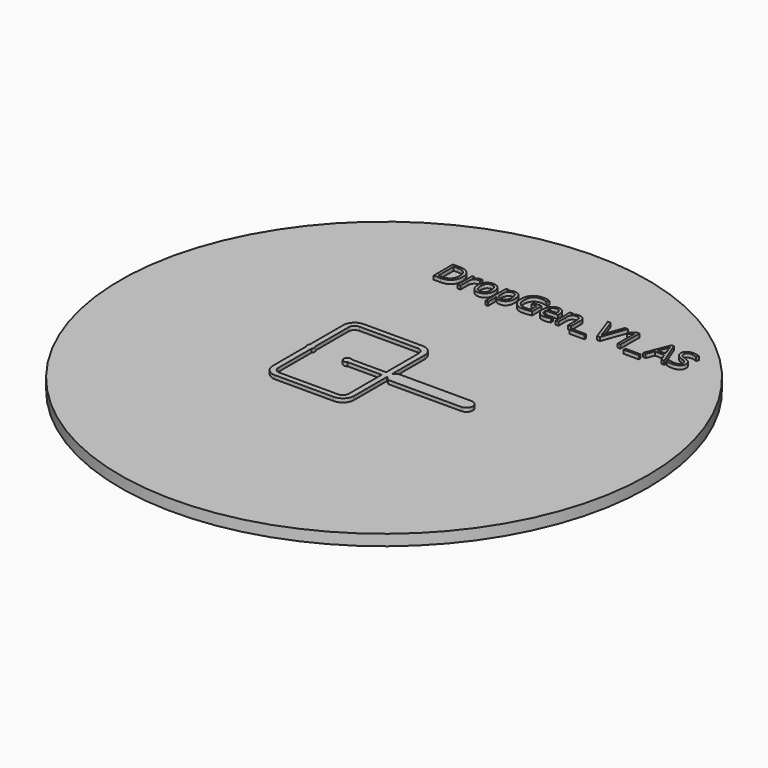
from build123d import *

# Parameters (mm, degrees)
F0_R         = 36
F0_W         = 2.0741813148
F0_H         = 0.2931375804
F0_TEXT_SIZE = 4.5869939236
F1_DEPTH     = 1.5
F2_DEPTH     = 0.5


# Not quite as in the source:
# - Text() gives the source's letters only with a copy of the font that has no kerning and outlines rounded to 1/6400 em; it was checked with that copy


with BuildPart() as f1:
    # F0 (on Top) → F1 (new body)
    with BuildSketch(Plane.XY):
        Circle(F0_R)
        with BuildLine():
            add(Edge.make_bspline(
                [(-6.0150917545, 23.3154267102), (-5.8222946662, 23.445510991), (-5.5915115344, 23.445510991)],
                knots=[0, 0, 0, 1, 1, 1], degree=2))
            add(Edge.make_bspline(
                [(-5.5915115344, 23.445510991), (-5.4280998758, 23.445510991), (-5.2983739539, 23.4182757146)],
                knots=[0, 0, 0, 1, 1, 1], degree=2))
            Line((-5.2983739539, 23.4182757146), (-5.3499776356, 23.0735344525))
            add(Edge.make_bspline(
                [(-5.3499776356, 23.0735344525), (-5.5019218093, 23.1072201892), (-5.6187468108, 23.1072201892)],
                knots=[0, 0, 0, 1, 1, 1], degree=2))
            add(Edge.make_bspline(
                [(-5.6187468108, 23.1072201892), (-5.9169014158, 23.1072201892), (-6.128333167, 22.8653279315)],
                knots=[0, 0, 0, 1, 1, 1], degree=2))
            add(Edge.make_bspline(
                [(-6.128333167, 22.8653279315), (-6.3397649182, 22.6234356738), (-6.3397649182, 22.2629266201)],
                knots=[0, 0, 0, 1, 1, 1], degree=2))
            Line((-6.3397649182, 22.2629266201), (-6.3397649182, 20.9455993026))
            Line((-6.3397649182, 20.9455993026), (-6.7117414567, 20.9455993026))
            Line((-6.7117414567, 20.9455993026), (-6.7117414567, 23.4003577696))
            Line((-6.7117414567, 23.4003577696), (-6.404986238, 23.4003577696))
            Line((-6.404986238, 23.4003577696), (-6.36198317, 22.945958684))
            Line((-6.36198317, 22.945958684), (-6.344065225, 22.945958684))
            add(Edge.make_bspline(
                [(-6.344065225, 22.945958684), (-6.2078888429, 23.1853424294), (-6.0150917545, 23.3154267102)],
                knots=[0, 0, 0, 1, 1, 1], degree=2))
        make_face(mode=Mode.SUBTRACT)
        with BuildLine():
            add(Edge.make_bspline(
                [(-3.0238700138, 23.1025615235), (-2.7203400253, 22.7596120559), (-2.7203400253, 22.1754870484)],
                knots=[0, 0, 0, 1, 1, 1], degree=2))
            add(Edge.make_bspline(
                [(-2.7203400253, 22.1754870484), (-2.7203400253, 21.5748775315), (-3.0224365782, 21.2376618064)],
                knots=[0, 0, 0, 1, 1, 1], degree=2))
            add(Edge.make_bspline(
                [(-3.0224365782, 21.2376618064), (-3.3245331312, 20.9004460812), (-3.8577711748, 20.9004460812)],
                knots=[0, 0, 0, 1, 1, 1], degree=2))
            add(Edge.make_bspline(
                [(-3.8577711748, 20.9004460812), (-4.1874613631, 20.9004460812), (-4.4426129001, 21.0552571261)],
                knots=[0, 0, 0, 1, 1, 1], degree=2))
            add(Edge.make_bspline(
                [(-4.4426129001, 21.0552571261), (-4.6977644371, 21.2100681711), (-4.8368076904, 21.4989054447)],
                knots=[0, 0, 0, 1, 1, 1], degree=2))
            add(Edge.make_bspline(
                [(-4.8368076904, 21.4989054447), (-4.9758509437, 21.7877427183), (-4.9758509437, 22.1754870484)],
                knots=[0, 0, 0, 1, 1, 1], degree=2))
            add(Edge.make_bspline(
                [(-4.9758509437, 22.1754870484), (-4.9758509437, 22.7753798475), (-4.6755461853, 23.1104454193)],
                knots=[0, 0, 0, 1, 1, 1], degree=2))
            add(Edge.make_bspline(
                [(-4.6755461853, 23.1104454193), (-4.3752414268, 23.445510991), (-3.8420033832, 23.445510991)],
                knots=[0, 0, 0, 1, 1, 1], degree=2))
            add(Edge.make_bspline(
                [(-3.8420033832, 23.445510991), (-3.3274000024, 23.445510991), (-3.0238700138, 23.1025615235)],
                knots=[0, 0, 0, 1, 1, 1], degree=2))
        make_face(mode=Mode.SUBTRACT)
        with BuildLine():
            add(Edge.make_bspline(
                [(-0.1763501922, 21.235511653), (-0.4461944441, 20.9004460812), (-0.9256786527, 20.9004460812)],
                knots=[0, 0, 0, 1, 1, 1], degree=2))
            add(Edge.make_bspline(
                [(-0.9256786527, 20.9004460812), (-1.1657791159, 20.9004460812), (-1.3639515877, 20.9889607296)],
                knots=[0, 0, 0, 1, 1, 1], degree=2))
            add(Edge.make_bspline(
                [(-1.3639515877, 20.9889607296), (-1.5621240596, 21.077475378), (-1.6961502883, 21.2616718527)],
                knots=[0, 0, 0, 1, 1, 1], degree=2))
            Line((-1.6961502883, 21.2616718527), (-1.7233855647, 21.2616718527))
            add(Edge.make_bspline(
                [(-1.7233855647, 21.2616718527), (-1.6961502883, 21.0466565125), (-1.6961502883, 20.8538594242)],
                knots=[0, 0, 0, 1, 1, 1], degree=2))
            Line((-1.6961502883, 20.8538594242), (-1.6961502883, 19.8432873254))
            Line((-1.6961502883, 19.8432873254), (-2.0681268268, 19.8432873254))
            Line((-2.0681268268, 19.8432873254), (-2.0681268268, 23.4003577696))
            Line((-2.0681268268, 23.4003577696), (-1.765671915, 23.4003577696))
            Line((-1.765671915, 23.4003577696), (-1.7140682333, 23.0642171211))
            Line((-1.7140682333, 23.0642171211), (-1.6961502883, 23.0642171211))
            add(Edge.make_bspline(
                [(-1.6961502883, 23.0642171211), (-1.5528067282, 23.2663315409), (-1.3625181521, 23.355921266)],
                knots=[0, 0, 0, 1, 1, 1], degree=2))
            add(Edge.make_bspline(
                [(-1.3625181521, 23.355921266), (-1.1722295761, 23.445510991), (-0.9256786527, 23.445510991)],
                knots=[0, 0, 0, 1, 1, 1], degree=2))
            add(Edge.make_bspline(
                [(-0.9256786527, 23.445510991), (-0.4375938305, 23.445510991), (-0.1720498854, 23.111520496)],
                knots=[0, 0, 0, 1, 1, 1], degree=2))
            add(Edge.make_bspline(
                [(-0.1720498854, 23.111520496), (0.0934940597, 22.7775300009), (0.0934940597, 22.1754870484)],
                knots=[0, 0, 0, 1, 1, 1], degree=2))
            add(Edge.make_bspline(
                [(0.0934940597, 22.1754870484), (0.0934940597, 21.5705772247), (-0.1763501922, 21.235511653)],
                knots=[0, 0, 0, 1, 1, 1], degree=2))
        make_face(mode=Mode.SUBTRACT)
        with BuildLine():
            add(Edge.make_bspline(
                [(-7.8093947682, 23.7970610722), (-7.386172907, 23.373839211), (-7.386172907, 22.6141183424)],
                knots=[0, 0, 0, 1, 1, 1], degree=2))
            add(Edge.make_bspline(
                [(-7.386172907, 22.6141183424), (-7.386172907, 21.8035105099), (-7.8262376365, 21.3745549063)],
                knots=[0, 0, 0, 1, 1, 1], degree=2))
            add(Edge.make_bspline(
                [(-7.8262376365, 21.3745549063), (-8.2663023661, 20.9455993026), (-9.0926779901, 20.9455993026)],
                knots=[0, 0, 0, 1, 1, 1], degree=2))
            Line((-9.0926779901, 20.9455993026), (-10.0000427257, 20.9455993026))
            Line((-10.0000427257, 20.9455993026), (-10.0000427257, 24.2202829334))
            Line((-10.0000427257, 24.2202829334), (-8.9966378049, 24.2202829334))
            add(Edge.make_bspline(
                [(-8.9966378049, 24.2202829334), (-8.2326166295, 24.2202829334), (-7.8093947682, 23.7970610722)],
                knots=[0, 0, 0, 1, 1, 1], degree=2))
        make_face(mode=Mode.SUBTRACT)
        with BuildLine():
            Line((-10.375, 0.3307189139), (-10.375, 6))
            ThreePointArc((-10.375, 6), (-9.9210155108, 7.0960155108), (-8.825, 7.55))
            Line((-8.825, 7.55), (-0.825, 7.55))
            ThreePointArc((-0.825, 7.55), (0.2710155108, 7.0960155108), (0.725, 6))
            Line((0.725, 6), (0.725, 0.375))
            Line((0.725, 0.375), (1.225, 0.875))
            Line((1.225, 0.875), (11.225, 0.875))
            ThreePointArc((11.225, 0.875), (11.8437184335, 0.6187184335), (12.1, 0))
            ThreePointArc((12.1, 0), (11.8437184335, -0.6187184335), (11.225, -0.875))
            Line((11.225, -0.875), (1.225, -0.875))
            Line((1.225, -0.875), (0.725, -0.375))
            Line((0.725, -0.375), (0.725, -6))
            ThreePointArc((0.725, -6), (0.2710155108, -7.0960155108), (-0.825, -7.55))
            Line((-0.825, -7.55), (-8.825, -7.55))
            ThreePointArc((-8.825, -7.55), (-9.9210155108, -7.0960155108), (-10.375, -6))
            Line((-10.375, -6), (-10.375, -0.3307189139))
            ThreePointArc((-10.375, -0.3307189139), (-10.5, 0), (-10.375, 0.3307189139))
        make_face(mode=Mode.SUBTRACT)
        with BuildLine():
            add(Edge.make_bspline(
                [(5.5434162152, 20.9377154068), (5.3678203541, 20.9004460812), (5.1191192773, 20.9004460812)],
                knots=[0, 0, 0, 1, 1, 1], degree=2))
            add(Edge.make_bspline(
                [(5.1191192773, 20.9004460812), (4.5751304666, 20.9004460812), (4.2601329933, 21.2322864229)],
                knots=[0, 0, 0, 1, 1, 1], degree=2))
            add(Edge.make_bspline(
                [(4.2601329933, 21.2322864229), (3.9451355199, 21.5641267645), (3.9451355199, 22.1525520788)],
                knots=[0, 0, 0, 1, 1, 1], degree=2))
            add(Edge.make_bspline(
                [(3.9451355199, 22.1525520788), (3.9451355199, 22.7467111355), (4.2375563826, 23.0961110632)],
                knots=[0, 0, 0, 1, 1, 1], degree=2))
            add(Edge.make_bspline(
                [(4.2375563826, 23.0961110632), (4.5299772452, 23.445510991), (5.023079092, 23.445510991)],
                knots=[0, 0, 0, 1, 1, 1], degree=2))
            add(Edge.make_bspline(
                [(5.023079092, 23.445510991), (5.4839286378, 23.445510991), (5.752697813, 23.1419810025)],
                knots=[0, 0, 0, 1, 1, 1], degree=2))
            add(Edge.make_bspline(
                [(5.752697813, 23.1419810025), (6.0214669882, 22.8384510139), (6.0214669882, 22.3410488604)],
                knots=[0, 0, 0, 1, 1, 1], degree=2))
            Line((6.0214669882, 22.3410488604), (6.0214669882, 22.1059654218))
            Line((6.0214669882, 22.1059654218), (4.3307296967, 22.1059654218))
            add(Edge.make_bspline(
                [(4.3307296967, 22.1059654218), (4.3421971815, 21.673784588), (4.5493286258, 21.4498102753)],
                knots=[0, 0, 0, 1, 1, 1], degree=2))
            add(Edge.make_bspline(
                [(4.5493286258, 21.4498102753), (4.7564600702, 21.2258359627), (5.1327369155, 21.2258359627)],
                knots=[0, 0, 0, 1, 1, 1], degree=2))
            add(Edge.make_bspline(
                [(5.1327369155, 21.2258359627), (5.5290818592, 21.2258359627), (5.9161094715, 21.3913977746)],
                knots=[0, 0, 0, 1, 1, 1], degree=2))
            Line((5.9161094715, 21.3913977746), (5.9161094715, 21.0595574329))
            add(Edge.make_bspline(
                [(5.9161094715, 21.0595574329), (5.7190120763, 20.9749847325), (5.5434162152, 20.9377154068)],
                knots=[0, 0, 0, 1, 1, 1], degree=2))
        make_face(mode=Mode.SUBTRACT)
        with BuildLine():
            Line((8.7077253047, 20.9455993026), (8.3357487662, 20.9455993026))
            Line((8.3357487662, 20.9455993026), (8.3357487662, 22.5338459487))
            add(Edge.make_bspline(
                [(8.3357487662, 22.5338459487), (8.3357487662, 22.8334339893), (8.1992140252, 22.9814362152)],
                knots=[0, 0, 0, 1, 1, 1], degree=2))
            add(Edge.make_bspline(
                [(8.1992140252, 22.9814362152), (8.0626792842, 23.129438441), (7.7709751394, 23.129438441)],
                knots=[0, 0, 0, 1, 1, 1], degree=2))
            add(Edge.make_bspline(
                [(7.7709751394, 23.129438441), (7.3860976805, 23.129438441), (7.2069182303, 22.9212319199)],
                knots=[0, 0, 0, 1, 1, 1], degree=2))
            add(Edge.make_bspline(
                [(7.2069182303, 22.9212319199), (7.0277387802, 22.7130253988), (7.0277387802, 22.2335411903)],
                knots=[0, 0, 0, 1, 1, 1], degree=2))
            Line((7.0277387802, 22.2335411903), (7.0277387802, 20.9455993026))
            Line((7.0277387802, 20.9455993026), (6.6557622417, 20.9455993026))
            Line((6.6557622417, 20.9455993026), (6.6557622417, 23.4003577696))
            Line((6.6557622417, 23.4003577696), (6.9582171535, 23.4003577696))
            Line((6.9582171535, 23.4003577696), (7.0184214488, 23.0642171211))
            Line((7.0184214488, 23.0642171211), (7.0363393938, 23.0642171211))
            add(Edge.make_bspline(
                [(7.0363393938, 23.0642171211), (7.1510142419, 23.2455467247), (7.3570706095, 23.3455288578)],
                knots=[0, 0, 0, 1, 1, 1], degree=2))
            add(Edge.make_bspline(
                [(7.3570706095, 23.3455288578), (7.5631269772, 23.445510991), (7.8161283608, 23.445510991)],
                knots=[0, 0, 0, 1, 1, 1], degree=2))
            add(Edge.make_bspline(
                [(7.8161283608, 23.445510991), (8.2597766793, 23.445510991), (8.483750992, 23.2315707276)],
                knots=[0, 0, 0, 1, 1, 1], degree=2))
            add(Edge.make_bspline(
                [(8.483750992, 23.2315707276), (8.7077253047, 23.0176304641), (8.7077253047, 22.5467468691)],
                knots=[0, 0, 0, 1, 1, 1], degree=2))
            Line((8.7077253047, 22.5467468691), (8.7077253047, 20.9455993026))
        make_face(mode=Mode.SUBTRACT)
        with BuildLine():
            Line((2.2393471546, 22.3209807619), (2.2393471546, 22.6614217172))
            Line((2.2393471546, 22.6614217172), (3.3524098989, 22.6614217172))
            Line((3.3524098989, 22.6614217172), (3.3524098989, 21.0688747643))
            add(Edge.make_bspline(
                [(3.3524098989, 21.0688747643), (3.0922413373, 20.9857354995), (2.8234721621, 20.9430907903)],
                knots=[0, 0, 0, 1, 1, 1], degree=2))
            add(Edge.make_bspline(
                [(2.8234721621, 20.9430907903), (2.5547029869, 20.9004460812), (2.2006443934, 20.9004460812)],
                knots=[0, 0, 0, 1, 1, 1], degree=2))
            add(Edge.make_bspline(
                [(2.2006443934, 20.9004460812), (1.4574080342, 20.9004460812), (1.0431451455, 21.3430193231)],
                knots=[0, 0, 0, 1, 1, 1], degree=2))
            add(Edge.make_bspline(
                [(1.0431451455, 21.3430193231), (0.6288822567, 21.7855925649), (0.6288822567, 22.5825827591)],
                knots=[0, 0, 0, 1, 1, 1], degree=2))
            add(Edge.make_bspline(
                [(0.6288822567, 22.5825827591), (0.6288822567, 23.0936025509), (0.8338635477, 23.477763292)],
                knots=[0, 0, 0, 1, 1, 1], degree=2))
            add(Edge.make_bspline(
                [(0.8338635477, 23.477763292), (1.0388448387, 23.8619240331), (1.4240806565, 24.0643968118)],
                knots=[0, 0, 0, 1, 1, 1], degree=2))
            add(Edge.make_bspline(
                [(1.4240806565, 24.0643968118), (1.8093164743, 24.2668695905), (2.3260700085, 24.2668695905)],
                knots=[0, 0, 0, 1, 1, 1], degree=2))
            add(Edge.make_bspline(
                [(2.3260700085, 24.2668695905), (2.8507074385, 24.2668695905), (3.3029563706, 24.0747892199)],
                knots=[0, 0, 0, 1, 1, 1], degree=2))
            Line((3.3029563706, 24.0747892199), (3.1553125037, 23.7386485715))
            add(Edge.make_bspline(
                [(3.1553125037, 23.7386485715), (2.7116641852, 23.9264286352), (2.3017016033, 23.9264286352)],
                knots=[0, 0, 0, 1, 1, 1], degree=2))
            add(Edge.make_bspline(
                [(2.3017016033, 23.9264286352), (1.7039589576, 23.9264286352), (1.3678183091, 23.5705782472)],
                knots=[0, 0, 0, 1, 1, 1], degree=2))
            add(Edge.make_bspline(
                [(1.3678183091, 23.5705782472), (1.0316776606, 23.2147278592), (1.0316776606, 22.5825827591)],
                knots=[0, 0, 0, 1, 1, 1], degree=2))
            add(Edge.make_bspline(
                [(1.0316776606, 22.5825827591), (1.0316776606, 21.9196187936), (1.3552757476, 21.5770276849)],
                knots=[0, 0, 0, 1, 1, 1], degree=2))
            add(Edge.make_bspline(
                [(1.3552757476, 21.5770276849), (1.6788738346, 21.2344365763), (2.3060019101, 21.2344365763)],
                knots=[0, 0, 0, 1, 1, 1], degree=2))
            add(Edge.make_bspline(
                [(2.3060019101, 21.2344365763), (2.6464428653, 21.2344365763), (2.971116029, 21.3132755343)],
                knots=[0, 0, 0, 1, 1, 1], degree=2))
            Line((2.971116029, 21.3132755343), (2.971116029, 22.3209807619))
            Line((2.971116029, 22.3209807619), (2.2393471546, 22.3209807619))
        make_face(mode=Mode.SUBTRACT)
        with Locations((10.104608298, 20.3869177771)):
            Rectangle(F0_W, F0_H, mode=Mode.SUBTRACT)
        with Locations((17.5133202024, 20.3869177771)):
            Rectangle(F0_W, F0_H, mode=Mode.SUBTRACT)
        with BuildLine():
            Line((12.7055771963, 22.1145660354), (13.45383058, 24.2202829334))
            Line((13.45383058, 24.2202829334), (13.8630764442, 24.2202829334))
            Line((13.8630764442, 24.2202829334), (12.6833589444, 20.9455993026))
            Line((12.6833589444, 20.9455993026), (12.3070820991, 20.9455993026))
            Line((12.3070820991, 20.9455993026), (11.1330983418, 24.2202829334))
            Line((11.1330983418, 24.2202829334), (11.5366104635, 24.2202829334))
            Line((11.5366104635, 24.2202829334), (12.2891641541, 22.101665115))
            add(Edge.make_bspline(
                [(12.2891641541, 22.101665115), (12.418890076, 21.7361390367), (12.4948621629, 21.3913977746)],
                knots=[0, 0, 0, 1, 1, 1], degree=2))
            add(Edge.make_bspline(
                [(12.4948621629, 21.3913977746), (12.5758512744, 21.7540569817), (12.7055771963, 22.1145660354)],
                knots=[0, 0, 0, 1, 1, 1], degree=2))
        make_face(mode=Mode.SUBTRACT)
        with BuildLine():
            Line((15.4642240106, 24.2202829334), (15.4642240106, 20.9455993026))
            Line((15.4642240106, 20.9455993026), (15.1015648035, 20.9455993026))
            Line((15.1015648035, 20.9455993026), (15.1015648035, 23.2792324613))
            add(Edge.make_bspline(
                [(15.1015648035, 23.2792324613), (15.1015648035, 23.5709366061), (15.1194827486, 23.8303884499)],
                knots=[0, 0, 0, 1, 1, 1], degree=2))
            add(Edge.make_bspline(
                [(15.1194827486, 23.8303884499), (15.0728960915, 23.7830850751), (15.0144835908, 23.7318397523)],
                knots=[0, 0, 0, 1, 1, 1], degree=2))
            add(Edge.make_bspline(
                [(15.0144835908, 23.7318397523), (14.95607109, 23.6805944296), (14.4816039061, 23.2950002529)],
                knots=[0, 0, 0, 1, 1, 1], degree=2))
            Line((14.4816039061, 23.2950002529), (14.2845065109, 23.5501517899))
            Line((14.2845065109, 23.5501517899), (15.1510183318, 24.2202829334))
            Line((15.1510183318, 24.2202829334), (15.4642240106, 24.2202829334))
        make_face(mode=Mode.SUBTRACT)
        Polygon((21.4445173385, 20.9455993026), (21.0503225482, 20.9455993026), (20.6425101197, 21.9869902669), (19.3301998269, 21.9869902669), (18.927404423, 20.9455993026), (18.5418102463, 20.9455993026), (19.8362025941, 24.2339005716), (20.1565754509, 24.2339005716), align=None, mode=Mode.SUBTRACT)
        with BuildLine():
            add(Edge.make_bspline(
                [(23.548800801, 22.3632671122), (23.7423146072, 22.1525520788), (23.7423146072, 21.8171281481)],
                knots=[0, 0, 0, 1, 1, 1], degree=2))
            add(Edge.make_bspline(
                [(23.7423146072, 21.8171281481), (23.7423146072, 21.3849473144), (23.4287505694, 21.1426966978)],
                knots=[0, 0, 0, 1, 1, 1], degree=2))
            add(Edge.make_bspline(
                [(23.4287505694, 21.1426966978), (23.1151865317, 20.9004460812), (22.5776481812, 20.9004460812)],
                knots=[0, 0, 0, 1, 1, 1], degree=2))
            add(Edge.make_bspline(
                [(22.5776481812, 20.9004460812), (21.9956733272, 20.9004460812), (21.6817509305, 21.0509568193)],
                knots=[0, 0, 0, 1, 1, 1], degree=2))
            Line((21.6817509305, 21.0509568193), (21.6817509305, 21.4179163332))
            add(Edge.make_bspline(
                [(21.6817509305, 21.4179163332), (21.8838653503, 21.3333436328), (22.1210989423, 21.2838901045)],
                knots=[0, 0, 0, 1, 1, 1], degree=2))
            add(Edge.make_bspline(
                [(22.1210989423, 21.2838901045), (22.3583325343, 21.2344365763), (22.5912658195, 21.2344365763)],
                knots=[0, 0, 0, 1, 1, 1], degree=2))
            add(Edge.make_bspline(
                [(22.5912658195, 21.2344365763), (22.9718429716, 21.2344365763), (23.1646400599, 21.3788552131)],
                knots=[0, 0, 0, 1, 1, 1], degree=2))
            add(Edge.make_bspline(
                [(23.1646400599, 21.3788552131), (23.3574371483, 21.5232738499), (23.3574371483, 21.7812922581)],
                knots=[0, 0, 0, 1, 1, 1], degree=2))
            add(Edge.make_bspline(
                [(23.3574371483, 21.7812922581), (23.3574371483, 21.9511543768), (23.2889905983, 22.0597371236)],
                knots=[0, 0, 0, 1, 1, 1], degree=2))
            add(Edge.make_bspline(
                [(23.2889905983, 22.0597371236), (23.2205440483, 22.1683198704), (23.0603576199, 22.2604181078)],
                knots=[0, 0, 0, 1, 1, 1], degree=2))
            add(Edge.make_bspline(
                [(23.0603576199, 22.2604181078), (22.9001711915, 22.3525163452), (22.5733478744, 22.4686246289)],
                knots=[0, 0, 0, 1, 1, 1], degree=2))
            add(Edge.make_bspline(
                [(22.5733478744, 22.4686246289), (22.1167986355, 22.6320362874), (21.920776317, 22.8560106001)],
                knots=[0, 0, 0, 1, 1, 1], degree=2))
            add(Edge.make_bspline(
                [(21.920776317, 22.8560106001), (21.7247539986, 23.0799849127), (21.7247539986, 23.4404939664)],
                knots=[0, 0, 0, 1, 1, 1], degree=2))
            add(Edge.make_bspline(
                [(21.7247539986, 23.4404939664), (21.7247539986, 23.8189209651), (22.0089326065, 24.0428952778)],
                knots=[0, 0, 0, 1, 1, 1], degree=2))
            add(Edge.make_bspline(
                [(22.0089326065, 24.0428952778), (22.2931112144, 24.2668695905), (22.761844656, 24.2668695905)],
                knots=[0, 0, 0, 1, 1, 1], degree=2))
            add(Edge.make_bspline(
                [(22.761844656, 24.2668695905), (23.2499294782, 24.2668695905), (23.6598920601, 24.0876901403)],
                knots=[0, 0, 0, 1, 1, 1], degree=2))
            Line((23.6598920601, 24.0876901403), (23.5409169052, 23.7565665165))
            add(Edge.make_bspline(
                [(23.5409169052, 23.7565665165), (23.1352546301, 23.9264286352), (22.7525273246, 23.9264286352)],
                knots=[0, 0, 0, 1, 1, 1], degree=2))
            add(Edge.make_bspline(
                [(22.7525273246, 23.9264286352), (22.4500724127, 23.9264286352), (22.2798519351, 23.7967027133)],
                knots=[0, 0, 0, 1, 1, 1], degree=2))
            add(Edge.make_bspline(
                [(22.2798519351, 23.7967027133), (22.1096314575, 23.6669767914), (22.1096314575, 23.4361936596)],
                knots=[0, 0, 0, 1, 1, 1], degree=2))
            add(Edge.make_bspline(
                [(22.1096314575, 23.4361936596), (22.1096314575, 23.2663315409), (22.172344265, 23.1573904352)],
                knots=[0, 0, 0, 1, 1, 1], degree=2))
            add(Edge.make_bspline(
                [(22.172344265, 23.1573904352), (22.2350570726, 23.0484493295), (22.3841343751, 22.9577845277)],
                knots=[0, 0, 0, 1, 1, 1], degree=2))
            add(Edge.make_bspline(
                [(22.3841343751, 22.9577845277), (22.5332116776, 22.867119726), (22.8399668962, 22.7574619025)],
                knots=[0, 0, 0, 1, 1, 1], degree=2))
            add(Edge.make_bspline(
                [(22.8399668962, 22.7574619025), (23.3552869949, 22.5739821455), (23.548800801, 22.3632671122)],
                knots=[0, 0, 0, 1, 1, 1], degree=2))
        make_face(mode=Mode.SUBTRACT)
        with BuildLine():
            ThreePointArc((-8.825, 7.55), (-9.9210155108, 7.0960155108), (-10.375, 6))
            Line((-10.375, 6), (-10.375, 0.3307189139))
            ThreePointArc((-10.375, 0.3307189139), (-10.5, 0), (-10.375, -0.3307189139))
            Line((-10.375, -0.3307189139), (-10.375, -6))
            ThreePointArc((-10.375, -6), (-9.9210155108, -7.0960155108), (-8.825, -7.55))
            Line((-8.825, -7.55), (-0.825, -7.55))
            ThreePointArc((-0.825, -7.55), (0.2710155108, -7.0960155108), (0.725, -6))
            Line((0.725, -6), (0.725, -0.375))
            Line((0.725, -0.375), (1.225, -0.875))
            Line((1.225, -0.875), (11.225, -0.875))
            ThreePointArc((11.225, -0.875), (10.35, 0), (11.225, 0.875))
            Line((11.225, 0.875), (1.225, 0.875))
            Line((1.225, 0.875), (0.725, 0.375))
            Line((0.725, 0.375), (0.725, 6))
            ThreePointArc((0.725, 6), (0.2710155108, 7.0960155108), (-0.825, 7.55))
            Line((-0.825, 7.55), (-8.825, 7.55))
        make_face()
        with BuildLine():
            Line((-9.625, 0.3307189139), (-9.625, 6))
            ThreePointArc((-9.625, 6), (-9.3906854249, 6.5656854249), (-8.825, 6.8))
            Line((-8.825, 6.8), (-0.825, 6.8))
            ThreePointArc((-0.825, 6.8), (-0.2593145751, 6.5656854249), (-0.025, 6))
            Line((-0.025, 6), (-0.025, 0.375))
            Line((-0.025, 0.375), (-4.6692810861, 0.375))
            ThreePointArc((-4.6692810861, 0.375), (-5.5, 0), (-4.6692810861, -0.375))
            Line((-4.6692810861, -0.375), (-0.025, -0.375))
            Line((-0.025, -0.375), (-0.025, -6))
            ThreePointArc((-0.025, -6), (-0.2593145751, -6.5656854249), (-0.825, -6.8))
            Line((-0.825, -6.8), (-8.825, -6.8))
            ThreePointArc((-8.825, -6.8), (-9.3906854249, -6.5656854249), (-9.625, -6))
            Line((-9.625, -6), (-9.625, -0.3307189139))
            ThreePointArc((-9.625, -0.3307189139), (-9.5, 0), (-9.625, 0.3307189139))
        make_face(mode=Mode.SUBTRACT)
        with BuildLine():
            ThreePointArc((-8.825, 6.8), (-9.3906854249, 6.5656854249), (-9.625, 6))
            Line((-9.625, 6), (-9.625, 0.3307189139))
            ThreePointArc((-9.625, 0.3307189139), (-9.5, 0), (-9.625, -0.3307189139))
            Line((-9.625, -0.3307189139), (-9.625, -6))
            ThreePointArc((-9.625, -6), (-9.3906854249, -6.5656854249), (-8.825, -6.8))
            Line((-8.825, -6.8), (-0.825, -6.8))
            ThreePointArc((-0.825, -6.8), (-0.2593145751, -6.5656854249), (-0.025, -6))
            Line((-0.025, -6), (-0.025, -0.375))
            Line((-0.025, -0.375), (-4.6692810861, -0.375))
            ThreePointArc((-4.6692810861, -0.375), (-5.5, 0), (-4.6692810861, 0.375))
            Line((-4.6692810861, 0.375), (-0.025, 0.375))
            Line((-0.025, 0.375), (-0.025, 6))
            ThreePointArc((-0.025, 6), (-0.2593145751, 6.5656854249), (-0.825, 6.8))
            Line((-0.825, 6.8), (-8.825, 6.8))
        make_face()
        with BuildLine():
            add(Edge.make_bspline(
                [(-8.1319177785, 21.6096383449), (-7.7889683109, 21.9447039166), (-7.7889683109, 22.6005007042)],
                knots=[0, 0, 0, 1, 1, 1], degree=2))
            add(Edge.make_bspline(
                [(-7.7889683109, 22.6005007042), (-7.7889683109, 23.2412464179), (-8.1104162445, 23.5659195815)],
                knots=[0, 0, 0, 1, 1, 1], degree=2))
            add(Edge.make_bspline(
                [(-8.1104162445, 23.5659195815), (-8.431864178, 23.8905927452), (-9.0661594315, 23.8905927452)],
                knots=[0, 0, 0, 1, 1, 1], degree=2))
            Line((-9.0661594315, 23.8905927452), (-9.6194655736, 23.8905927452))
            Line((-9.6194655736, 23.8905927452), (-9.6194655736, 21.2745727731))
            Line((-9.6194655736, 21.2745727731), (-9.1557491566, 21.2745727731))
            add(Edge.make_bspline(
                [(-9.1557491566, 21.2745727731), (-8.474867246, 21.2745727731), (-8.1319177785, 21.6096383449)],
                knots=[0, 0, 0, 1, 1, 1], degree=2))
        make_face()
        with BuildLine():
            ThreePointArc((12.1, 0), (11.8437184335, 0.6187184335), (11.225, 0.875))
            ThreePointArc((11.225, 0.875), (10.35, 0), (11.225, -0.875))
            ThreePointArc((11.225, -0.875), (11.8437184335, -0.6187184335), (12.1, 0))
        make_face()
        with BuildLine():
            add(Edge.make_bspline(
                [(-4.4042684977, 22.8896963367), (-4.590256767, 22.6499542324), (-4.590256767, 22.1754870484)],
                knots=[0, 0, 0, 1, 1, 1], degree=2))
            add(Edge.make_bspline(
                [(-4.590256767, 22.1754870484), (-4.590256767, 21.7046034534), (-4.4021183443, 21.458410889)],
                knots=[0, 0, 0, 1, 1, 1], degree=2))
            add(Edge.make_bspline(
                [(-4.4021183443, 21.458410889), (-4.2139799217, 21.2122183245), (-3.8491705612, 21.2122183245)],
                knots=[0, 0, 0, 1, 1, 1], degree=2))
            add(Edge.make_bspline(
                [(-3.8491705612, 21.2122183245), (-3.4836444829, 21.2122183245), (-3.2944309836, 21.4573358123)],
                knots=[0, 0, 0, 1, 1, 1], degree=2))
            add(Edge.make_bspline(
                [(-3.2944309836, 21.4573358123), (-3.1052174842, 21.7024533), (-3.1052174842, 22.1754870484)],
                knots=[0, 0, 0, 1, 1, 1], degree=2))
            add(Edge.make_bspline(
                [(-3.1052174842, 22.1754870484), (-3.1052174842, 22.6435037722), (-3.2944309836, 22.8864711066)],
                knots=[0, 0, 0, 1, 1, 1], degree=2))
            add(Edge.make_bspline(
                [(-3.2944309836, 22.8864711066), (-3.4836444829, 23.129438441), (-3.853470868, 23.129438441)],
                knots=[0, 0, 0, 1, 1, 1], degree=2))
            add(Edge.make_bspline(
                [(-3.853470868, 23.129438441), (-4.2182802285, 23.129438441), (-4.4042684977, 22.8896963367)],
                knots=[0, 0, 0, 1, 1, 1], degree=2))
        make_face()
        with BuildLine():
            add(Edge.make_bspline(
                [(-0.4723546438, 22.8843209532), (-0.6526091707, 23.129438441), (-0.9794324877, 23.129438441)],
                knots=[0, 0, 0, 1, 1, 1], degree=2))
            add(Edge.make_bspline(
                [(-0.9794324877, 23.129438441), (-1.355709333, 23.129438441), (-1.5237796573, 22.9212319199)],
                knots=[0, 0, 0, 1, 1, 1], degree=2))
            add(Edge.make_bspline(
                [(-1.5237796573, 22.9212319199), (-1.6918499815, 22.7130253988), (-1.6961502883, 22.2579095955)],
                knots=[0, 0, 0, 1, 1, 1], degree=2))
            Line((-1.6961502883, 22.2579095955), (-1.6961502883, 22.1754870484))
            add(Edge.make_bspline(
                [(-1.6961502883, 22.1754870484), (-1.6961502883, 21.6580167964), (-1.5237796573, 21.4351175604)],
                knots=[0, 0, 0, 1, 1, 1], degree=2))
            add(Edge.make_bspline(
                [(-1.5237796573, 21.4351175604), (-1.3514090262, 21.2122183245), (-0.9708318741, 21.2122183245)],
                knots=[0, 0, 0, 1, 1, 1], degree=2))
            add(Edge.make_bspline(
                [(-0.9708318741, 21.2122183245), (-0.6526091707, 21.2122183245), (-0.4723546438, 21.4698783738)],
                knots=[0, 0, 0, 1, 1, 1], degree=2))
            add(Edge.make_bspline(
                [(-0.4723546438, 21.4698783738), (-0.292100117, 21.7275384231), (-0.292100117, 22.1797873552)],
                knots=[0, 0, 0, 1, 1, 1], degree=2))
            add(Edge.make_bspline(
                [(-0.292100117, 22.1797873552), (-0.292100117, 22.6392034654), (-0.4723546438, 22.8843209532)],
                knots=[0, 0, 0, 1, 1, 1], degree=2))
        make_face()
        with BuildLine():
            Line((19.4649427734, 22.3295813755), (20.5242516826, 22.3295813755))
            Line((20.5242516826, 22.3295813755), (20.1429578127, 23.3444537811))
            add(Edge.make_bspline(
                [(20.1429578127, 23.3444537811), (20.0691358793, 23.5372508695), (19.991013639, 23.8167708117)],
                knots=[0, 0, 0, 1, 1, 1], degree=2))
            add(Edge.make_bspline(
                [(19.991013639, 23.8167708117), (19.9415601108, 23.6017554715), (19.8498202323, 23.3444537811)],
                knots=[0, 0, 0, 1, 1, 1], degree=2))
            Line((19.8498202323, 23.3444537811), (19.4649427734, 22.3295813755))
        make_face()
        with BuildLine():
            add(Edge.make_bspline(
                [(5.4663690516, 22.9466754018), (5.3097662122, 23.1337387478), (5.0180620674, 23.1337387478)],
                knots=[0, 0, 0, 1, 1, 1], degree=2))
            add(Edge.make_bspline(
                [(5.0180620674, 23.1337387478), (4.7227743336, 23.1337387478), (4.5468201135, 22.9413000183)],
                knots=[0, 0, 0, 1, 1, 1], degree=2))
            add(Edge.make_bspline(
                [(4.5468201135, 22.9413000183), (4.3708658935, 22.7488612889), (4.3393303103, 22.4084203336)],
                knots=[0, 0, 0, 1, 1, 1], degree=2))
            Line((4.3393303103, 22.4084203336), (5.6229718911, 22.4084203336))
            add(Edge.make_bspline(
                [(5.6229718911, 22.4084203336), (5.6229718911, 22.7596120559), (5.4663690516, 22.9466754018)],
                knots=[0, 0, 0, 1, 1, 1], degree=2))
        make_face()
        with Locations((-10.4501415044, 20.9455993026)):
            Text('DropGen_V1_AS', F0_TEXT_SIZE, font='Open Sans', text_align=(TextAlign.LEFT, TextAlign.BOTTOM))
    extrude(amount=-F1_DEPTH)

    # F0 (on Top) → F2 (join)
    with BuildSketch(Plane.XY):
        with BuildLine():
            ThreePointArc((-8.825, 7.55), (-9.9210155108, 7.0960155108), (-10.375, 6))
            Line((-10.375, 6), (-10.375, 0.3307189139))
            ThreePointArc((-10.375, 0.3307189139), (-10.5, 0), (-10.375, -0.3307189139))
            Line((-10.375, -0.3307189139), (-10.375, -6))
            ThreePointArc((-10.375, -6), (-9.9210155108, -7.0960155108), (-8.825, -7.55))
            Line((-8.825, -7.55), (-0.825, -7.55))
            ThreePointArc((-0.825, -7.55), (0.2710155108, -7.0960155108), (0.725, -6))
            Line((0.725, -6), (0.725, -0.375))
            Line((0.725, -0.375), (1.225, -0.875))
            Line((1.225, -0.875), (11.225, -0.875))
            ThreePointArc((11.225, -0.875), (10.35, 0), (11.225, 0.875))
            Line((11.225, 0.875), (1.225, 0.875))
            Line((1.225, 0.875), (0.725, 0.375))
            Line((0.725, 0.375), (0.725, 6))
            ThreePointArc((0.725, 6), (0.2710155108, 7.0960155108), (-0.825, 7.55))
            Line((-0.825, 7.55), (-8.825, 7.55))
        make_face()
        with BuildLine():
            Line((-9.625, 0.3307189139), (-9.625, 6))
            ThreePointArc((-9.625, 6), (-9.3906854249, 6.5656854249), (-8.825, 6.8))
            Line((-8.825, 6.8), (-0.825, 6.8))
            ThreePointArc((-0.825, 6.8), (-0.2593145751, 6.5656854249), (-0.025, 6))
            Line((-0.025, 6), (-0.025, 0.375))
            Line((-0.025, 0.375), (-4.6692810861, 0.375))
            ThreePointArc((-4.6692810861, 0.375), (-5.5, 0), (-4.6692810861, -0.375))
            Line((-4.6692810861, -0.375), (-0.025, -0.375))
            Line((-0.025, -0.375), (-0.025, -6))
            ThreePointArc((-0.025, -6), (-0.2593145751, -6.5656854249), (-0.825, -6.8))
            Line((-0.825, -6.8), (-8.825, -6.8))
            ThreePointArc((-8.825, -6.8), (-9.3906854249, -6.5656854249), (-9.625, -6))
            Line((-9.625, -6), (-9.625, -0.3307189139))
            ThreePointArc((-9.625, -0.3307189139), (-9.5, 0), (-9.625, 0.3307189139))
        make_face(mode=Mode.SUBTRACT)
        with BuildLine():
            ThreePointArc((12.1, 0), (11.8437184335, 0.6187184335), (11.225, 0.875))
            ThreePointArc((11.225, 0.875), (10.35, 0), (11.225, -0.875))
            ThreePointArc((11.225, -0.875), (11.8437184335, -0.6187184335), (12.1, 0))
        make_face()
        with Locations((-10.4501415044, 20.9455993026)):
            Text('DropGen_V1_AS', F0_TEXT_SIZE, font='Open Sans', text_align=(TextAlign.LEFT, TextAlign.BOTTOM))
    extrude(amount=F2_DEPTH)


solid = f1.part
